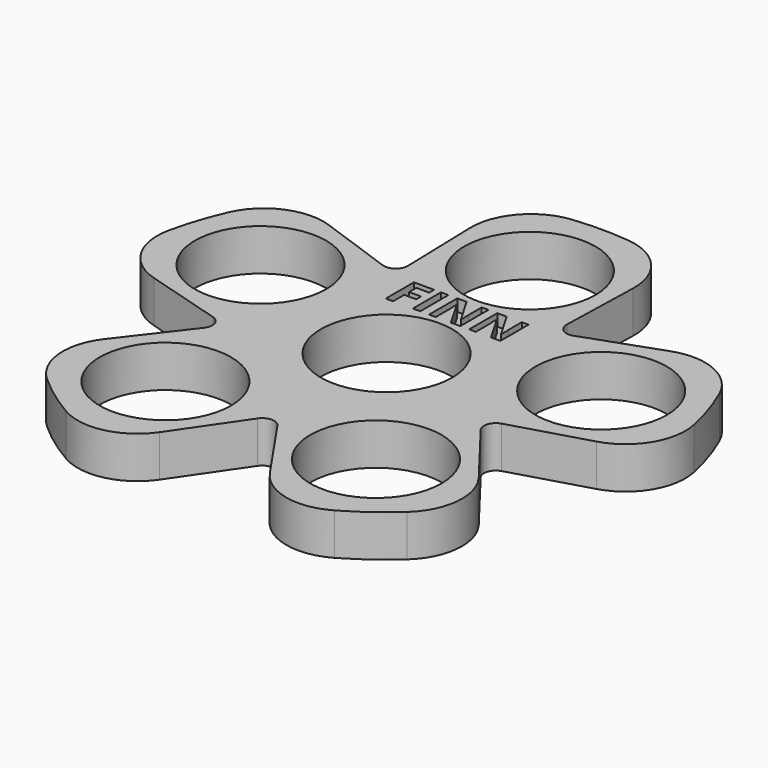
from build123d import *

# Parameters (mm, degrees)
F0_R         = 45
F0_R_2       = 11
F1_DEPTH     = 7
F3_DEPTH     = 25
F4_R         = 10
F5_R         = 2
F6_TEXT_SIZE = 8.2527688291
F7_DEPTH     = 2


# Not quite as in the source:
# - Text() gives the source's letters only with a copy of the font that has no kerning and outlines rounded to 1/6400 em; it was checked with that copy


with BuildPart() as f1:
    # F0 (on Top) → F1 (new body)
    with BuildSketch(Plane.XY):
        Circle(F0_R)
        with Locations((-17.6335575688, -24.2705098312)):
            Circle(F0_R_2, mode=Mode.SUBTRACT)
        with Locations((17.6335575688, -24.2705098312)):
            Circle(F0_R_2, mode=Mode.SUBTRACT)
        with Locations((-28.5316954889, 9.2705098312)):
            Circle(F0_R_2, mode=Mode.SUBTRACT)
        Circle(F0_R_2, mode=Mode.SUBTRACT)
        with Locations((28.5316954889, 9.2705098312)):
            Circle(F0_R_2, mode=Mode.SUBTRACT)
        with Locations((0, 30)):
            Circle(F0_R_2, mode=Mode.SUBTRACT)
    extrude(amount=F1_DEPTH)

    # F2 (on face) → F3 (cut)
    with BuildSketch(Plane.XY.offset(7)):
        with BuildLine():
            Line((-13.2251681766, 18.2028823734), (-13.9057647469, 42.7975432333))
            ThreePointArc((-13.9057647469, 42.7975432333), (-26.4503363532, 36.4057647469), (-36.4057647469, 26.4503363532))
            Line((-36.4057647469, 26.4503363532), (-13.2251681766, 18.2028823734))
        make_face()
        with BuildLine():
            ThreePointArc((36.4057647469, 26.4503363532), (26.4503363532, 36.4057647469), (13.9057647469, 42.7975432333))
            Line((13.9057647469, 42.7975432333), (13.2251681766, 18.2028823734))
            Line((13.2251681766, 18.2028823734), (36.4057647469, 26.4503363532))
        make_face()
        with BuildLine():
            ThreePointArc((36.4057647469, -26.4503363532), (42.7975432333, -13.9057647469), (45, 0))
            Line((45, 0), (21.3987716166, -6.9528823734))
            Line((21.3987716166, -6.9528823734), (36.4057647469, -26.4503363532))
        make_face()
        with BuildLine():
            ThreePointArc((-13.9057647469, -42.7975432333), (0, -45), (13.9057647469, -42.7975432333))
            Line((13.9057647469, -42.7975432333), (0, -22.5))
            Line((0, -22.5), (-13.9057647469, -42.7975432333))
        make_face()
        with BuildLine():
            Line((-21.3987716166, -6.9528823734), (-45, 0))
            ThreePointArc((-45, 0), (-42.7975432333, -13.9057647469), (-36.4057647469, -26.4503363532))
            Line((-36.4057647469, -26.4503363532), (-21.3987716166, -6.9528823734))
        make_face()
    extrude(amount=-F3_DEPTH, mode=Mode.SUBTRACT)

    # F4
    f4_edges = [f1.edges().sort_by_distance(p)[0] for p in [
        (45, 0, 3.5),
        (36.405765, 26.450336, 3.5),
        (36.405765, -26.450336, 3.5),
        (13.905765, -42.797543, 3.5),
        (-13.905765, -42.797543, 3.5),
        (-36.405765, -26.450336, 3.5),
        (-45, 0, 3.5),
        (-36.405765, 26.450336, 3.5),
        (-13.905765, 42.797543, 3.5),
        (13.905765, 42.797543, 3.5),
    ]]
    fillet(f4_edges, radius=F4_R)

    # F5
    f5_edges = [f1.edges().sort_by_distance(p)[0] for p in [
        (13.225168, 18.202882, 3.5),
        (21.398772, -6.952882, 3.5),
        (0, -22.5, 3.5),
        (-21.398772, -6.952882, 3.5),
        (-13.225168, 18.202882, 3.5),
    ]]
    fillet(f5_edges, radius=F5_R)

    # F6 (on face) → F7 (cut)
    with BuildSketch(Plane.XY.offset(7)):
        with Locations((-10.5233278591, 12.0613900945)):
            Text('FINN', F6_TEXT_SIZE, font='Open Sans', font_style=FontStyle.BOLD, text_align=(TextAlign.LEFT, TextAlign.BOTTOM))
    extrude(amount=-F7_DEPTH, mode=Mode.SUBTRACT)


solid = f1.part
